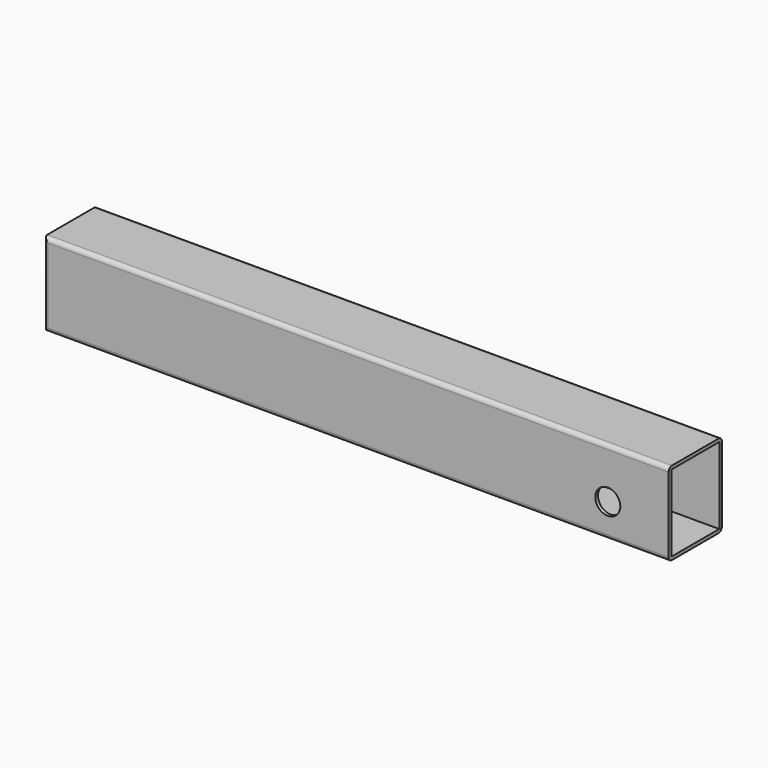
from build123d import *

# Parameters (mm, degrees)
F1_DEPTH     = 80
F2_T         = 4
F3_T1_DEPTH  = 774.9998275448
F3_T3_DEPTH  = 124.9996550895
F3_T6_ANGLE  = 90.0000000944
F3_T8_ANGLE  = 89.9999999363
F3_T10_ANGLE = 90.0000000944
F3_T12_ANGLE = 89.9999999363
F4_R         = 15
F5_DEPTH     = 80.001


# Not quite as in the source:
# - a fillet or chamfer that OpenCascade refuses, or shapes differently, is made with other operations: its cross-section is extruded or revolved along the edge and cut away or added
# - a shell that OpenCascade refuses in one call is made with other operations: the cavity is built on its own and cut out


with BuildPart() as f1:
    # F0 (on Front) → F1 (new body)
    with BuildSketch(Plane.XZ):
        with BuildLine():
            Line((-374.9998275448, -50), (375, -50))
            Line((375, -50), (375, 50))
            Line((375, 50), (-374.9998275448, 50))
            ThreePointArc((-374.9998275448, 50), (-374.999949489, 49.999949489), (-375, 49.9998275448))
            Line((-375, 49.9998275448), (-375, -49.9998275448))
            ThreePointArc((-375, -49.9998275448), (-374.999949489, -49.999949489), (-374.9998275448, -50))
        make_face()
    extrude(amount=F1_DEPTH)

    # F2: shell of thickness 4, made by hand


with BuildPart() as f2_core1:
    # F2_t2: copy of F1
    add(f1.part)

    # the walls: a layer under each face that stays
    f2_faces = [f2_core1.faces().sort_by_distance(p)[0] for p in [
        (8.62276e-05, -40, -50),
        (8.62276e-05, -40, 50),
        (0, 0, 0),
        (0, -80, 0),
    ]]
    thicken(f2_faces, amount=-F2_T, mode=Mode.SUBTRACT)


with BuildPart() as f1_1:
    add(f1.part)

    # what is left inside the walls is the cavity
    f2_cavity = [f2_core1.part.solids().sort_by_distance(p)[0] for p in [
        (0, -4.04, -16.666667),
    ]]
    add(f2_cavity, mode=Mode.SUBTRACT)

    # F3: fillet of radius 5 on 4 edges, made by hand

    # F3_s2 → F3_t1 (cut)
    with BuildSketch(Plane.YZ.offset(-387.4998275448)):
        with BuildLine():
            ThreePointArc((-80, 45), (-78.5355339059, 48.5355339059), (-75, 50))
            Line((-75, 50), (-80, 50))
            Line((-80, 50), (-80, 45))
        make_face()
        with BuildLine():
            ThreePointArc((0, 45), (-1.4644660941, 48.5355339059), (-5, 50))
            Line((-5, 50), (0, 50))
            Line((0, 50), (0, 45))
        make_face()
        with BuildLine():
            ThreePointArc((-5, -50), (-1.4644660941, -48.5355339059), (0, -45))
            Line((0, -45), (0, -50))
            Line((0, -50), (-5, -50))
        make_face()
        with BuildLine():
            ThreePointArc((-75, -50), (-78.5355339059, -48.5355339059), (-80, -45))
            Line((-80, -45), (-80, -50))
            Line((-80, -50), (-75, -50))
        make_face()
    extrude(amount=F3_T1_DEPTH, mode=Mode.SUBTRACT)

    # F3_s4 → F3_t3 (cut)
    with BuildSketch(Plane.XY.offset(-62.4998275448)):
        with BuildLine():
            ThreePointArc((-370, -80), (-373.5355339059, -78.5355339059), (-375, -75))
            Line((-375, -75), (-375, -80))
            Line((-375, -80), (-370, -80))
        make_face()
        with BuildLine():
            ThreePointArc((-370, 0), (-373.5355339059, -1.4644660941), (-375, -5))
            Line((-375, -5), (-375, 0))
            Line((-375, 0), (-370, 0))
        make_face()
    extrude(amount=F3_T3_DEPTH, mode=Mode.SUBTRACT)

    # F3_s5 → F3_t6 (revolve, cut)
    with BuildSketch(Plane.XY.offset(-49.9998275448)):
        with BuildLine():
            ThreePointArc((-375, -75), (-374.999956886, -75.0207638646), (-374.9998275448, -75.0415273711))
            Line((-374.9998275448, -75.0415273711), (-374.9998275448, -80))
            Line((-374.9998275448, -80), (-375, -80))
            Line((-375, -80), (-375, -75))
        make_face()
    revolve(axis=Axis((-374.9998275448, -80, -49.9998275448), (0, -1, 0)), revolution_arc=F3_T6_ANGLE, mode=Mode.SUBTRACT)

    # F3_s7 → F3_t8 (revolve, cut)
    with BuildSketch(Plane.YZ.offset(-374.9998275448)):
        with BuildLine():
            ThreePointArc((-75.0415273711, 49.9998275448), (-75.0207638646, 49.999956886), (-75, 50))
            Line((-75, 50), (-80, 50))
            Line((-80, 50), (-80, 49.9998275448))
            Line((-80, 49.9998275448), (-75.0415273711, 49.9998275448))
        make_face()
    revolve(axis=Axis((-374.9998275448, -80, 49.9998275448), (0, -1, 0)), revolution_arc=F3_T8_ANGLE, mode=Mode.SUBTRACT)

    # F3_s9 → F3_t10 (revolve, cut)
    with BuildSketch(Plane.XY.offset(-49.9998275448)):
        with BuildLine():
            ThreePointArc((-375, -5), (-374.999956886, -4.9792361354), (-374.9998275448, -4.9584726289))
            Line((-374.9998275448, -4.9584726289), (-374.9998275448, 0))
            Line((-374.9998275448, 0), (-375, 0))
            Line((-375, 0), (-375, -5))
        make_face()
    revolve(axis=Axis((-374.9998275448, 0, -49.9998275448), (0, -1, 0)), revolution_arc=F3_T10_ANGLE, mode=Mode.SUBTRACT)

    # F3_s11 → F3_t12 (revolve, cut)
    with BuildSketch(Plane.YZ.offset(-374.9998275448)):
        with BuildLine():
            ThreePointArc((-4.9584726289, 49.9998275448), (-4.9792361354, 49.999956886), (-5, 50))
            Line((-5, 50), (0, 50))
            Line((0, 50), (0, 49.9998275448))
            Line((0, 49.9998275448), (-4.9584726289, 49.9998275448))
        make_face()
    revolve(axis=Axis((-374.9998275448, 0, 49.9998275448), (0, -1, 0)), revolution_arc=F3_T12_ANGLE, mode=Mode.SUBTRACT)

    # F4 (on Front) → F5 (cut, through all)
    with BuildSketch(Plane.XZ):
        with Locations((302, -10)):
            Circle(F4_R)
    extrude(amount=F5_DEPTH, mode=Mode.SUBTRACT)


solid = f1_1.part
